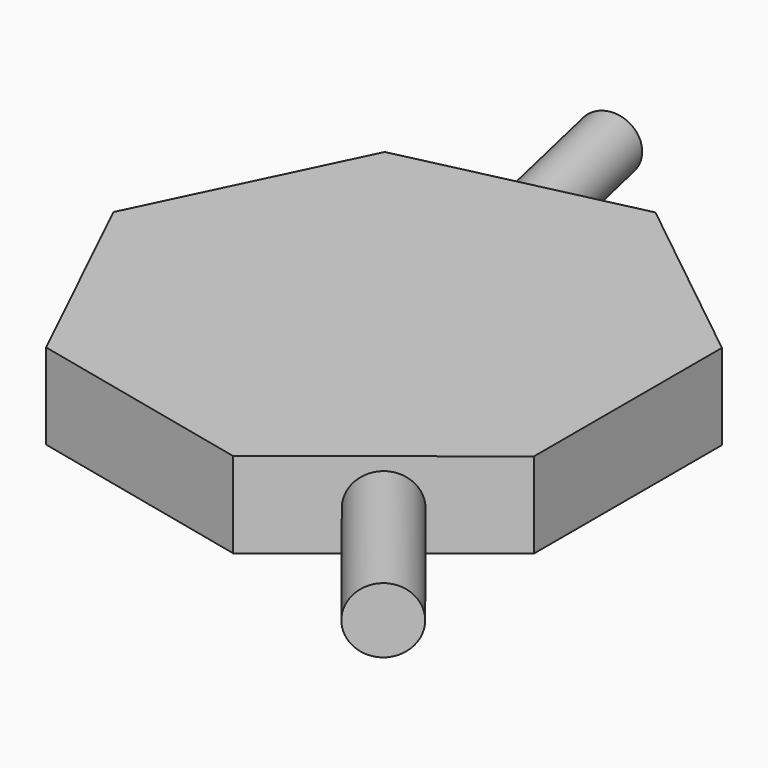
from build123d import *

# Parameters (mm, degrees)
F1_DEPTH = 25.4
F2_R     = 9.7144872298
F3_DEPTH = 56.2097504735
F4_R     = 8.5689068518
F5_DEPTH = 47.313503921


with BuildPart() as f1:
    # F0 (on Top) → F1 (new body)
    with BuildSketch(Plane.XY):
        Polygon((72.3621845245, -34.8477914285), (72.3621845245, 34.8477914285), (17.871983658, 78.3022765744), (-50.076185425, 62.7935503844), (-80.315965515, 0), (-50.076185425, -62.7935503844), (17.871983658, -78.3022765744), align=None)
    extrude(amount=F1_DEPTH)

    # F2 (on face) → F3 (join)
    with BuildSketch(Plane(origin=(45.1170840913, -56.5750340014, 0), x_dir=(0.7818314825, 0.6234898019, 0), z_dir=(0.6234898019, -0.7818314825, 0))):
        with Locations((0, 11.8007967249)):
            Circle(F2_R)
    extrude(amount=F3_DEPTH)

    # F4 (on face) → F5 (join)
    with BuildSketch(Plane(origin=(-16.1021008835, 70.5479134794, 0), x_dir=(-0.9749279122, -0.222520934, 0), z_dir=(-0.222520934, 0.9749279122, 0))):
        with Locations((0, 13.1539618596)):
            Circle(F4_R)
    extrude(amount=F5_DEPTH)


solid = f1.part
